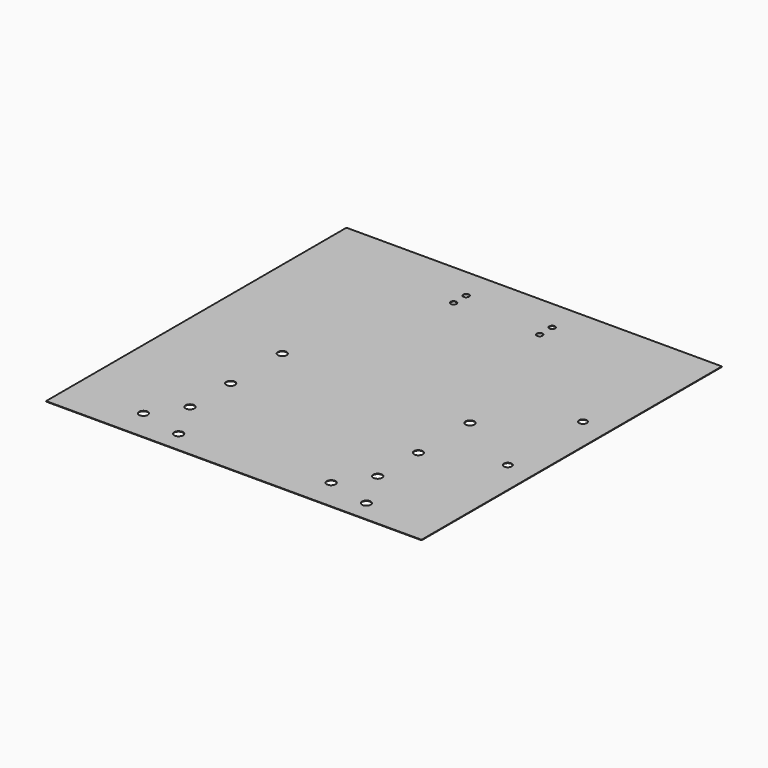
from build123d import *

# Parameters (mm, degrees)
F0_W     = 609.6
F0_H     = 609.6
F1_DEPTH = 0.79375
F2_R     = 7.14375
F3_DEPTH = 25.4
F4_R     = 4.7625
F5_DEPTH = 25.4
F6_R     = 6.35
F7_DEPTH = 25.4


# Not quite as in the source:
# - a feature names something its author has since deleted; it is built from what else it names


with BuildPart() as f1:
    # F0 (on Top) → F1 (new body)
    with BuildSketch(Plane.XY):
        with Locations((304.8, 304.8)):
            Rectangle(F0_W, F0_H)
    extrude(amount=F1_DEPTH)

    # F2 (on face) → F3 (cut)
    with BuildSketch(Plane.XY.offset(0.79375)):
        with Locations((187.325, 34.925)):
            Circle(F2_R)
        with Locations((117.475, 50.8)):
            Circle(F2_R)
        with Locations((152.4, 101.6)):
            Circle(F2_R)
        with Locations((152.4, 184.15)):
            Circle(F2_R)
        with Locations((152.4, 288.925)):
            Circle(F2_R)
        with Locations((457.2, 288.925)):
            Circle(F2_R)
        with Locations((457.2, 184.15)):
            Circle(F2_R)
        with Locations((457.2, 101.6)):
            Circle(F2_R)
        with Locations((422.275, 50.8)):
            Circle(F2_R)
        with Locations((492.125, 34.925)):
            Circle(F2_R)
    extrude(amount=-F3_DEPTH, mode=Mode.SUBTRACT)

    # F4 (on face) → F5 (cut)
    with BuildSketch(Plane.XY.offset(0.79375)):
        with Locations((234.95, 558.8)):
            Circle(F4_R)
        with Locations((234.95, 533.4)):
            Circle(F4_R)
        with Locations((374.65, 533.4)):
            Circle(F4_R)
        with Locations((374.65, 558.8)):
            Circle(F4_R)
    extrude(amount=-F5_DEPTH, mode=Mode.SUBTRACT)

    # F6 (on face) → F7 (cut)
    with BuildSketch(Plane(origin=(0, 0, 0), x_dir=(1, 0, 0), z_dir=(0, 0, -1))):
        with Locations((566.7375, -381)):
            Circle(F6_R)
        with Locations((566.7375, -228.6)):
            Circle(F6_R)
    extrude(amount=-F7_DEPTH, mode=Mode.SUBTRACT)


solid = f1.part
